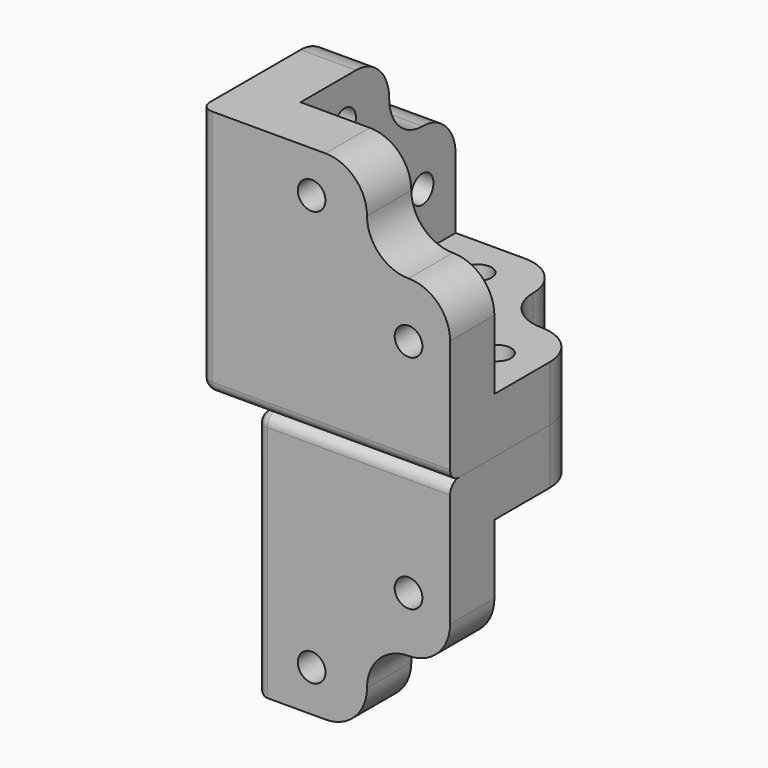
from build123d import *

# Parameters (mm, degrees)
F0_R      = 2.5
F1_DEPTH  = 10
F2_R      = 2.5
F3_DEPTH  = 10
F4_R      = 2.5
F5_DEPTH  = 10
F6_R      = 2
F7_R      = 7.5
F8_R      = 7.49999
F10_R     = 2.5
F11_DEPTH = 10
F12_R     = 2


# Not quite as in the source:
# - a fillet or chamfer is up to 0.001 mm smaller than in the source, because OpenCascade refuses the exact size
# - a feature names something its author has since deleted; it is built from what else it names


with BuildPart() as f1:
    # F0 (on Top) → F1 (new body)
    with BuildSketch(Plane.XY):
        Polygon((10, 10), (10, 45), (0, 45), (0, 0), (45, 0), (45, 10), align=None)
        Polygon((30, 45), (10, 45), (10, 10), (45, 10), (45, 30), (30, 30), align=None)
        with Locations((37.5, 20)):
            Circle(F0_R, mode=Mode.SUBTRACT)
        with Locations((20, 37.5)):
            Circle(F0_R, mode=Mode.SUBTRACT)
    extrude(amount=F1_DEPTH)

    # F2 (on Right) → F3 (join)
    with BuildSketch(Plane.YZ):
        Polygon((10, 10), (10, 45), (0, 45), (0, 0), (45, 0), (45, 10), align=None)
        Polygon((30, 45), (10, 45), (10, 10), (45, 10), (45, 30), (30, 30), align=None)
        with Locations((37.5, 20)):
            Circle(F2_R, mode=Mode.SUBTRACT)
        with Locations((20, 37.5)):
            Circle(F2_R, mode=Mode.SUBTRACT)
    extrude(amount=F3_DEPTH)

    # F4 (on Front) → F5 (join)
    with BuildSketch(Plane.XZ):
        Polygon((10, 10), (10, 45), (0, 45), (0, 0), (45, 0), (45, 10), align=None)
        Polygon((30, 45), (10, 45), (10, 10), (45, 10), (45, 30), (30, 30), align=None)
        with Locations((37.5, 20)):
            Circle(F4_R, mode=Mode.SUBTRACT)
        with Locations((20, 37.5)):
            Circle(F4_R, mode=Mode.SUBTRACT)
    extrude(amount=-F5_DEPTH)

    # F6
    f6_edges = [f1.edges().sort_by_distance(p)[0] for p in [
        (22.5, 0, 0),
        (0, 0, 22.5),
        (0, 22.5, 0),
    ]]
    fillet(f6_edges, radius=F6_R)

    # F7
    f7_edges = [f1.edges().sort_by_distance(p)[0] for p in [
        (45, 5, 30),
        (30, 5, 45),
        (5, 30, 45),
        (5, 45, 30),
        (30, 45, 5),
        (45, 30, 5),
    ]]
    fillet(f7_edges, radius=F7_R)

    # F8 (radius 7.5 in the source; OpenCascade refuses exactly that, so slightly less here)
    f8_edges = [f1.edges().sort_by_distance(p)[0] for p in [
        (30, 5, 30),
        (30, 30, 5),
        (5, 30, 30),
    ]]
    fillet(f8_edges, radius=F8_R)


with BuildPart() as f9_1:
    # F9: instance of F1
    add(f1.part.mirror(Plane.XY))

    # F10 (on face) → F11 (cut, through all)
    with BuildSketch(Plane(origin=(0, 0, 0), x_dir=(0, -1, 0), z_dir=(-1, 0, 0))):
        with BuildLine():
            Line((-45, -2), (-45, -22.5))
            ThreePointArc((-45, -22.5), (-42.8033008589, -27.8033008589), (-37.5, -30))
            ThreePointArc((-37.5, -30), (-32.1966991411, -32.1966991411), (-30, -37.5))
            ThreePointArc((-30, -37.5), (-27.8033008589, -42.8033008589), (-22.5, -45))
            Line((-22.5, -45), (-2, -45))
            Line((-2, -45), (-2, -2))
            Line((-2, -2), (-45, -2))
        make_face()
        with Locations((-20, -37.5)):
            Circle(F10_R, mode=Mode.SUBTRACT)
        with Locations((-37.5, -20)):
            Circle(F10_R, mode=Mode.SUBTRACT)
        with BuildLine():
            Line((-45, 0), (-45, -2))
            Line((-45, -2), (-2, -2))
            Line((-2, -2), (-2, -45))
            Line((-2, -45), (0, -45))
            Line((0, -45), (0, -37.5))
            Line((0, -37.5), (0, -30))
            Line((0, -30), (0, -22.5))
            Line((0, -22.5), (0, -2))
            ThreePointArc((0, -2), (-0.5857864376, -0.5857864376), (-2, 0))
            Line((-2, 0), (-45, 0))
        make_face()
    extrude(amount=-F11_DEPTH, mode=Mode.SUBTRACT)

    # F12
    f12_edges = [f9_1.edges().sort_by_distance(p)[0] for p in [
        (10, 45, -5),
        (10, 23.5, 0),
        (10, 0.585786, -0.585786),
        (10, 0, -23.5),
        (10, 5, -45),
        (10, 10, -27.5),
        (10, 27.5, -10),
    ]]
    fillet(f12_edges, radius=F12_R)


solid = Compound([f1.part, f9_1.part])
